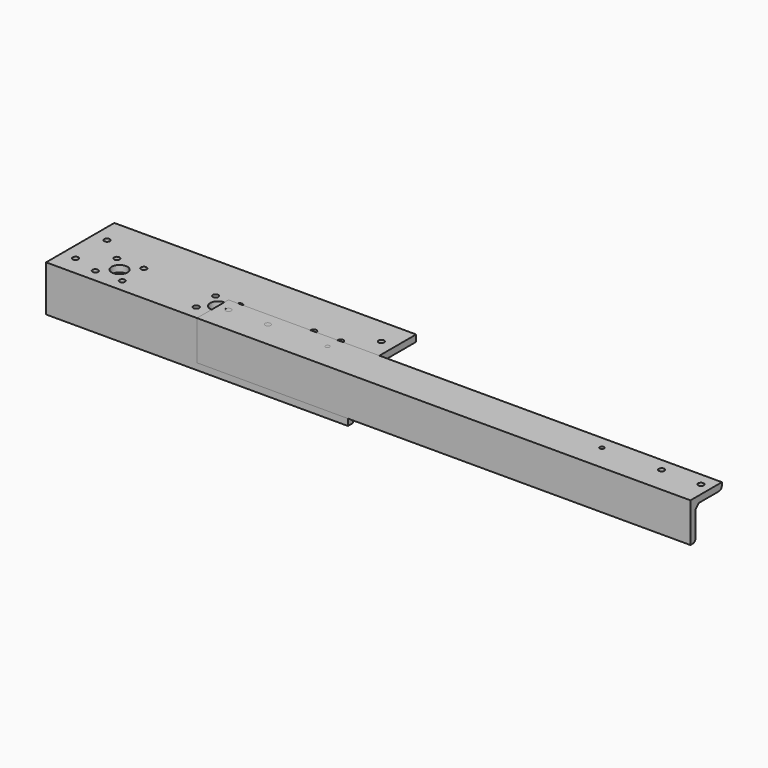
from build123d import *

# Parameters (mm, degrees)
F4_DEPTH  = 115
F6_R      = 6
F6_R_2    = 2.15
F8_DEPTH  = 25
F7_R      = 6
F7_R_2    = 2.15
F9_DEPTH  = 25
F10_DEPTH = 376
F11_R     = 2.15
F12_DEPTH = 25
F13_R     = 2.15
F14_DEPTH = 25
F15_R     = 1.6
F16_DEPTH = 25


with BuildPart() as f4:
    # F0 (on Right) → F4 (new body, symmetric)
    with BuildSketch(Plane.YZ):
        Polygon((0, 0), (0, -35), (5, -35), (5, -5), (65, -5), (65, 0), align=None)
    extrude(amount=F4_DEPTH, both=True)

    # F6 (on face) → F8 (cut)
    with BuildSketch(Plane.XY):
        with Locations((0, 20)):
            Circle(F6_R)
        with Locations((9.1923881554, 29.1923881554)):
            Circle(F6_R_2)
        with Locations((-9.1923881554, 29.1923881554)):
            Circle(F6_R_2)
        with Locations((-9.1923881554, 10.8076118446)):
            Circle(F6_R_2)
        with Locations((9.1923881554, 10.8076118446)):
            Circle(F6_R_2)
    extrude(amount=-F8_DEPTH, mode=Mode.SUBTRACT)

    # F7 (on face) → F9 (cut)
    with BuildSketch(Plane.XY):
        with Locations((-75, 20)):
            Circle(F7_R)
        with Locations((-64.7469516728, 30.2530483272)):
            Circle(F7_R_2)
        with Locations((-85.2530483272, 30.2530483272)):
            Circle(F7_R_2)
        with Locations((-85.2530483272, 9.7469516728)):
            Circle(F7_R_2)
        with Locations((-64.7469516728, 9.7469516728)):
            Circle(F7_R_2)
        with Locations((64.7469516728, 9.7469516728)):
            Circle(F7_R_2)
        with Locations((85.2530483272, 9.7469516728)):
            Circle(F7_R_2)
        with Locations((85.2530483272, 30.2530483272)):
            Circle(F7_R_2)
        with Locations((64.7469516728, 30.2530483272)):
            Circle(F7_R_2)
        with Locations((75, 20)):
            Circle(F7_R)
    extrude(amount=-F9_DEPTH, mode=Mode.SUBTRACT)

    # F11 (on face) → F12 (cut)
    with BuildSketch(Plane.XY):
        with Locations((-104.5, 45)):
            Circle(F11_R)
        with Locations((-104.5, 15)):
            Circle(F11_R)
        with Locations((104.5, 45)):
            Circle(F11_R)
        with Locations((104.5, 15)):
            Circle(F11_R)
    extrude(amount=-F12_DEPTH, mode=Mode.SUBTRACT)


with BuildPart() as f10:
    # F1 (on Right) → F10 (new body)
    with BuildSketch(Plane.YZ):
        with BuildLine():
            Line((0, 0), (0, -30))
            Line((0, -30), (2, -30))
            ThreePointArc((2, -30), (4.1213203436, -29.1213203436), (5, -27))
            Line((5, -27), (5, -8))
            Line((5, -8), (5, -5))
            Line((5, -5), (8, -5))
            Line((8, -5), (27, -5))
            ThreePointArc((27, -5), (29.1213203436, -4.1213203436), (30, -2))
            Line((30, -2), (30, 0))
            Line((30, 0), (0, 0))
        make_face()
        Polygon((5, -5), (5, -8), (8, -5), align=None)
    extrude(amount=F10_DEPTH)

    # F13 (on face) → F14 (cut)
    with BuildSketch(Plane.XY):
        with Locations((8, 20)):
            Circle(F13_R)
        with Locations((38, 20)):
            Circle(F13_R)
        with Locations((368, 20)):
            Circle(F13_R)
        with Locations((338, 20)):
            Circle(F13_R)
    extrude(amount=-F14_DEPTH, mode=Mode.SUBTRACT)

    # F15 (on face) → F16 (cut)
    with BuildSketch(Plane.XY):
        with Locations((83.5, 20)):
            Circle(F15_R)
        with Locations((292.5, 20)):
            Circle(F15_R)
    extrude(amount=-F16_DEPTH, mode=Mode.SUBTRACT)


solid = Compound([f4.part, f10.part])
